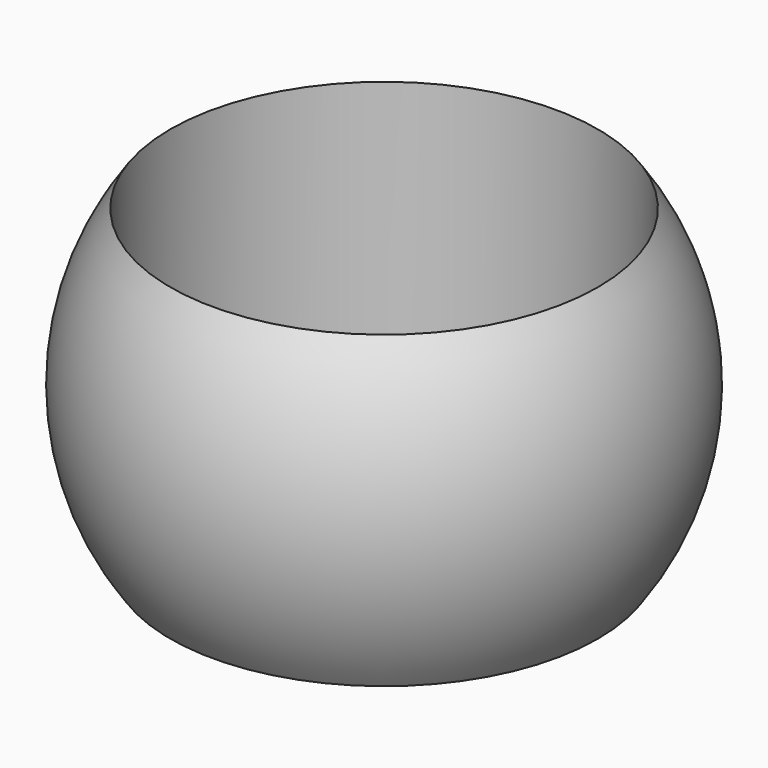
from build123d import *

# Parameters (mm, degrees)
F5_R     = 25.9345729703
F6_DEPTH = 176.9


# Not quite as in the source:
# - the program builds the solid bodies; features that only make, move or delete a surface that nothing else refers to are left out


with BuildPart() as f2:
    # F1 (on Front) → F2 (revolve)
    with BuildSketch(Plane.XZ):
        with BuildLine():
            Line((0, -32.0114270779), (0, 32.0114270779))
            ThreePointArc((0, 32.0114270779), (-32.0114270779, 0), (0, -32.0114270779))
        make_face()
    revolve(axis=Axis((0, 0, 0), (0, 0, -1)))

    # F5 (on offset) → F6 (cut)
    with BuildSketch(Plane.XY.offset(-56.8)):
        Circle(F5_R)
    extrude(amount=F6_DEPTH, mode=Mode.SUBTRACT)


solid = f2.part
